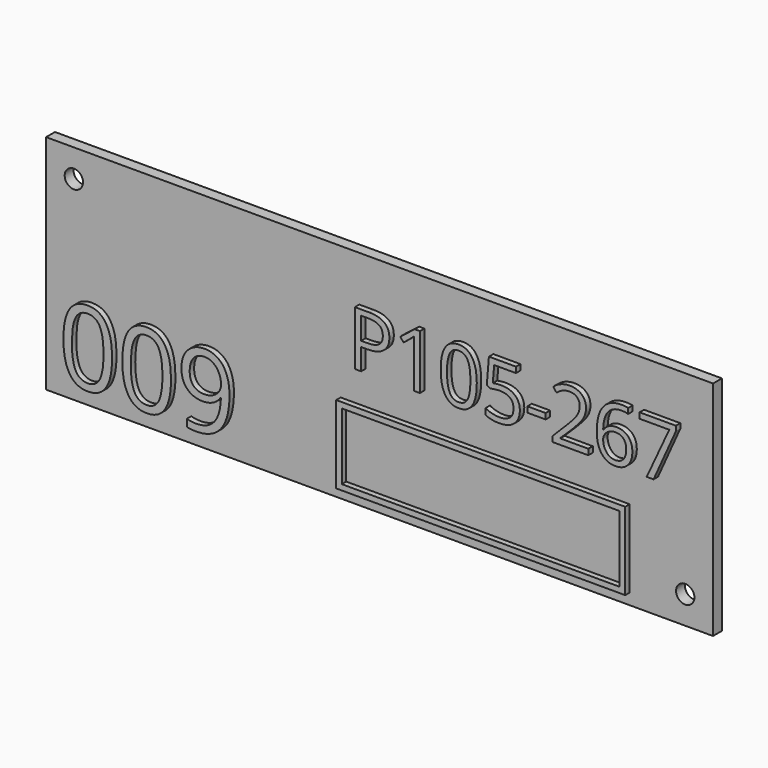
from build123d import *

# Parameters (mm, degrees)
F0_W         = 120
F0_H         = 40
F1_DEPTH     = 2
F3_D         = 3.3
F4_TEXT_SIZE = 13.7358706539
F5_DEPTH     = 1
F6_TEXT_SIZE = 18.5356140827
F7_DEPTH     = 1
F8_W         = 52
F8_H         = 14
F8_W_2       = 49.99999962
F8_H_2       = 11.99999962
F9_DEPTH     = 1


# Not quite as in the source:
# - Text() gives the source's letters only with a copy of the font that has no kerning and outlines rounded to 1/6400 em; it was checked with that copy


with BuildPart() as f1:
    # F0 (on Front) → F1 (new body)
    with BuildSketch(Plane.XZ):
        Rectangle(F0_W, F0_H)
    extrude(amount=F1_DEPTH)

    # F3 (through all)
    with Locations(Plane.XZ.offset(2)):
        with Locations((-55, 15), (55, -15)):
            Hole(F3_D / 2)

    # F4 (on face) → F5 (join)
    with BuildSketch(Plane.XZ.offset(2)):
        with Locations((-5, 2)):
            Text('P105-267', F4_TEXT_SIZE, font='Open Sans', text_align=(TextAlign.LEFT, TextAlign.BOTTOM))
    extrude(amount=F5_DEPTH)

    # F6 (on face) → F7 (join)
    with BuildSketch(Plane.XZ.offset(2)):
        with Locations((-57, -17)):
            Text('009', F6_TEXT_SIZE, font='Open Sans', text_align=(TextAlign.LEFT, TextAlign.BOTTOM))
    extrude(amount=F7_DEPTH)

    # F8 (on face) → F9 (join)
    with BuildSketch(Plane.XZ.offset(2)):
        with Locations((19, -11)):
            Rectangle(F8_W, F8_H)
        with Locations((19, -11)):
            Rectangle(F8_W_2, F8_H_2, mode=Mode.SUBTRACT)
    extrude(amount=F9_DEPTH)


solid = f1.part
